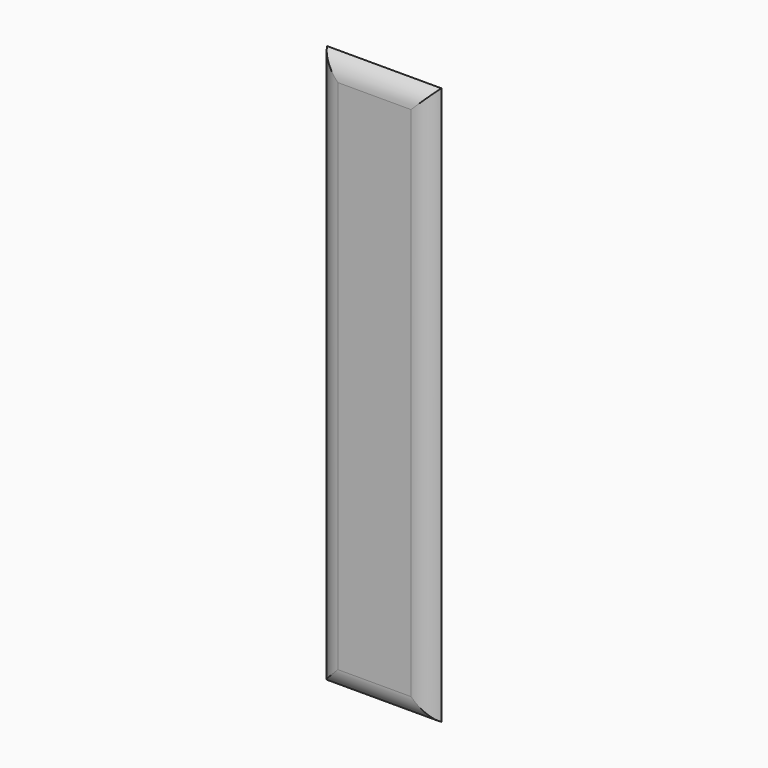
from build123d import *

# Parameters (mm, degrees)
F0_W        = 23.9217849086
F0_H        = 116.84
F1_DEPTH    = 2.54
F2_T1_DEPTH = 45.4097259166
F2_T3_DEPTH = 138.3279410079


# Not quite as in the source:
# - a fillet or chamfer that OpenCascade refuses, or shapes differently, is made with other operations: its cross-section is extruded or revolved along the edge and cut away or added


with BuildPart() as f1:
    # F0 (on Front) → F1 (new body)
    with BuildSketch(Plane.XZ):
        with Locations((-36.8977272883, -44.3508948228)):
            Rectangle(F0_W, F0_H)
    extrude(amount=F1_DEPTH)

    # F2: fillet of radius 4.9056819587 on 4 edges, made by hand

    # F2_s2 → F2_t1 (cut)
    with BuildSketch(Plane.YZ.offset(-59.6025902466)):
        with BuildLine():
            ThreePointArc((0, 14.0691051772), (-1.8575276492, 12.267557057), (-2.54, 9.7715169756))
            Line((-2.54, 9.7715169756), (-2.54, 14.0691051772))
            Line((-2.54, 14.0691051772), (0, 14.0691051772))
        make_face()
        with BuildLine():
            ThreePointArc((0, -102.7708948228), (-1.8575276492, -100.9693467025), (-2.54, -98.4733066212))
            Line((-2.54, -98.4733066212), (-2.54, -102.7708948228))
            Line((-2.54, -102.7708948228), (0, -102.7708948228))
        make_face()
    extrude(amount=F2_T1_DEPTH, mode=Mode.SUBTRACT)

    # F2_s4 → F2_t3 (cut)
    with BuildSketch(Plane.XY.offset(-113.5148653268)):
        with BuildLine():
            ThreePointArc((-48.8586197426, 0), (-47.0570716224, -1.8575276492), (-44.561031541, -2.54))
            Line((-44.561031541, -2.54), (-48.8586197426, -2.54))
            Line((-48.8586197426, -2.54), (-48.8586197426, 0))
        make_face()
        with BuildLine():
            ThreePointArc((-24.936834834, 0), (-26.7383829542, -1.8575276492), (-29.2344230356, -2.54))
            Line((-29.2344230356, -2.54), (-24.936834834, -2.54))
            Line((-24.936834834, -2.54), (-24.936834834, 0))
        make_face()
    extrude(amount=F2_T3_DEPTH, mode=Mode.SUBTRACT)


solid = f1.part
